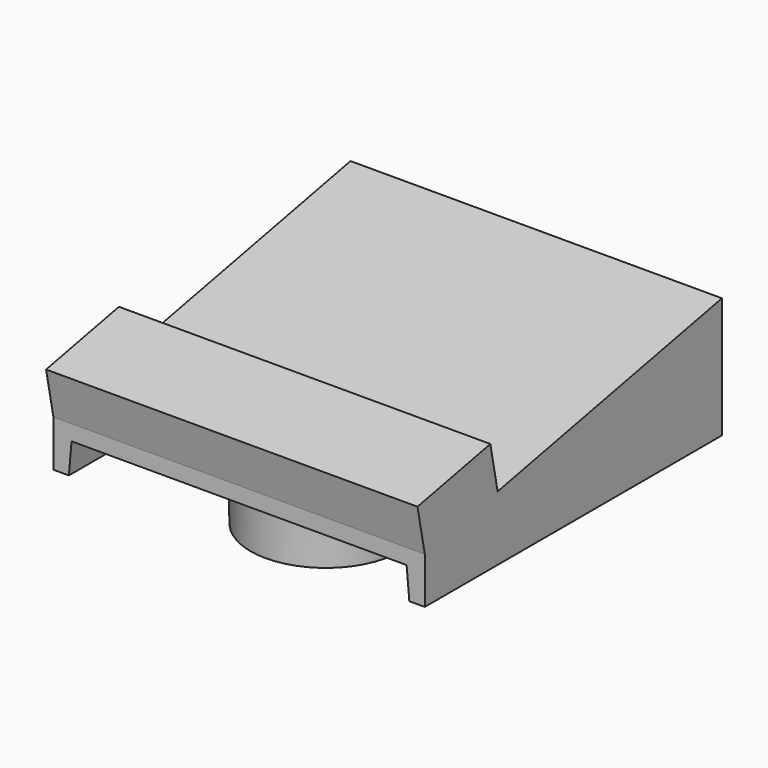
from build123d import *

# Parameters (mm, degrees)
F0_W                   = 152.4
F0_H                   = 152.4
F1_DEPTH               = 6.35
F3_DEPTH               = 152.4
F5_DEPTH               = 152.4
F7_DEPTH               = 25.4
DRAFT_F7_DRAFTED_ANGLE = 2


# Not quite as in the source:
# - an extrude with a draft is written as a straight extrude whose walls are then drafted


with BuildPart() as f1:
    # F0 (on Top) → F1 (new body)
    with BuildSketch(Plane.XY):
        Rectangle(F0_W, F0_H)
    extrude(amount=F1_DEPTH)

    # F2 (on face) → F3 (join, through all)
    with BuildSketch(Plane(origin=(-76.2, 0, 0), x_dir=(0, -1, 0), z_dir=(-1, 0, 0))):
        Polygon((-76.2, 6.35), (76.2, 6.35), (38.8409430132, 13.8273565556), (-76.2, 36.852620542), align=None)
        Polygon((38.8409430132, 13.8273565556), (76.2, 6.35), (79.9386782778, 25.0295284934), (42.579621291, 32.506885049), align=None)
    extrude(amount=-F3_DEPTH)

    # F4 (on face) → F5 (join, through all)
    with BuildSketch(Plane.XZ.offset(76.2)):
        Polygon((-68.7388939732, 0), (-76.2, 0), (-76.2, -12.7), (-69.85, -12.7), align=None)
        Polygon((76.2, 0), (68.7388939732, 0), (69.85, -12.7), (76.2, -12.7), align=None)
    extrude(amount=-F5_DEPTH)


with BuildPart() as f7_drafted:
    # F6 (on face) → F7 (new body)
    with BuildSketch(Plane(origin=(0, 0, 0), x_dir=(1, 0, 0), z_dir=(0, 0, -1))):
        with BuildLine():
            ThreePointArc((-17.2965677992, 5.1249884062), (15.1475488508, 3.8463395983), (31.75, 31.75))
            ThreePointArc((31.75, 31.75), (-9.260774135, 62.1194017462), (-26.3476732233, 14.0338317993))
            ThreePointArc((-26.3476732233, 14.0338317993), (-22.2721084825, 9.1222364397), (-17.2965677992, 5.1249884062))
        make_face()
        with BuildLine():
            ThreePointArc((-17.2965677992, 5.1249884062), (-22.2721084825, 9.1222364397), (-26.3476732233, 14.0338317993))
            Line((-26.3476732233, 14.0338317993), (-40.1609262841, 0))
            ThreePointArc((-40.1609262841, 0), (-40.0897952686, -8.9799744086), (-31.10982086, -8.908843393))
            Line((-31.10982086, -8.908843393), (-17.2965677992, 5.1249884062))
        make_face()
    extrude(amount=F7_DEPTH)

    # draft_F7_drafted
    draft_f7_drafted_walls = [f7_drafted.faces().sort_by_distance(p)[0] for p in [
        (22.2721084825, -54.3777635603, -16.9333333333),
        (-33.2542997537, -7.0169158996, -16.9333333333),
        (-40.0897952686, 8.9799744086, -16.9333333333),
        (-24.2031943296, 1.8919274934, -16.9333333333),
    ]]
    draft(draft_f7_drafted_walls, neutral_plane=Plane(origin=(0, 0, 0), x_dir=(1, 0, 0), z_dir=(0, 0, -1)), angle=DRAFT_F7_DRAFTED_ANGLE)


with BuildPart() as f1_1:
    add(f1.part)

    # join_F7_drafted: union F7_drafted
    add(f7_drafted.part)


solid = f1_1.part
